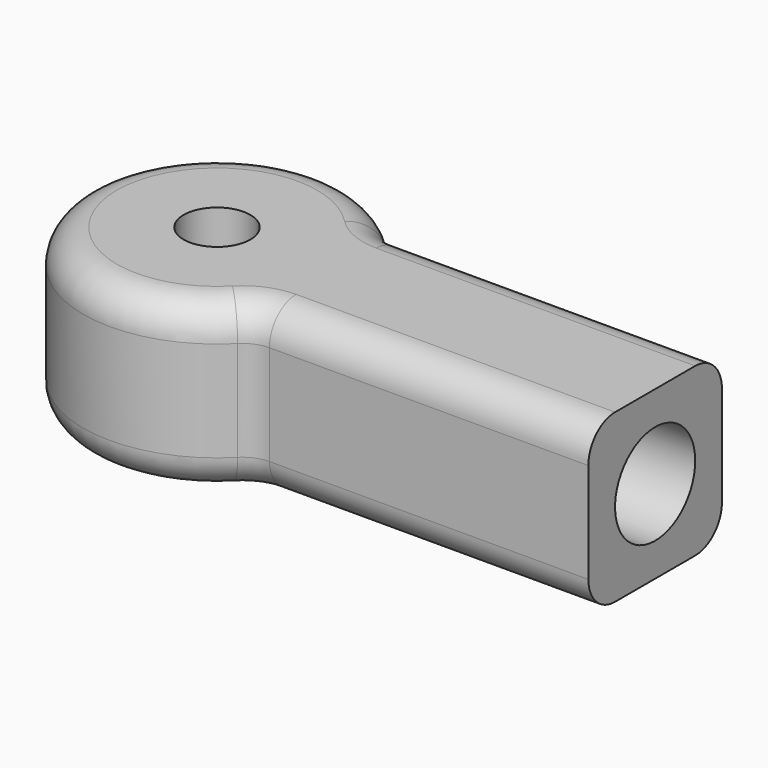
from build123d import *

# Parameters (mm, degrees)
F0_R     = 1
F1_DEPTH = 5
F2_R     = 1.5
F3_DEPTH = 10
F4_F1_R  = 1
F4_F2_R  = 1


with BuildPart() as f1:
    # F0 (on Top) → F1 (new body)
    with BuildSketch(Plane.XY):
        with BuildLine():
            Line((13.1224989992, 2.5), (3.1224989992, 2.5))
            ThreePointArc((3.1224989992, 2.5), (-4, 0), (3.1224989992, -2.5))
            Line((3.1224989992, -2.5), (13.1224989992, -2.5))
            Line((13.1224989992, -2.5), (13.1224989992, 2.5))
        make_face()
        Circle(F0_R, mode=Mode.SUBTRACT)
    extrude(amount=F1_DEPTH)

    # F2 (on face) → F3 (cut)
    with BuildSketch(Plane.YZ.offset(13.1224989992)):
        with Locations((0, 2.5)):
            Circle(F2_R)
    extrude(amount=-F3_DEPTH, mode=Mode.SUBTRACT)

    # F4: fillet of radius 1 on 4 edges, made by hand

    # F4_f1
    f4_f1_edges = [f1.edges().sort_by_distance(p)[0] for p in [
        (3.1224989992, 2.5, 2.5),
        (3.1224989992, -2.5, 2.5),
    ]]
    fillet(f4_f1_edges, radius=F4_F1_R)

    # F4_f2
    f4_f2_edges = [f1.edges().sort_by_distance(p)[0] for p in [
        (8.3466066067, -2.5, 5),
        (8.3466066067, -2.5, 0),
        (3.1834158797, -2.5780455543, 0),
        (3.1834158797, -2.5780455543, 5),
    ]]
    fillet(f4_f2_edges, radius=F4_F2_R)


solid = f1.part
